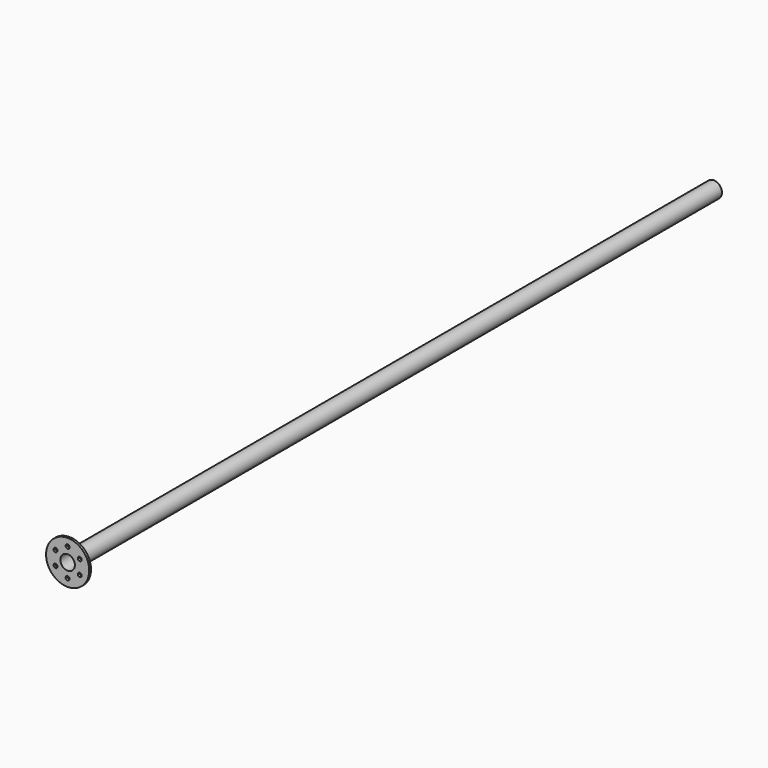
from build123d import *

# Parameters (mm, degrees)
F0_R            = 18.25
F0_R_2          = 16.25
F1_DEPTH        = 1800
F2_R            = 48.25
F2_R_2          = 18.25
F2_R_3          = 16.25
F3_DEPTH        = 5
F5_D            = 8.8
F5_COPIES_COUNT = 6


# Not quite as in the source:
# - a pattern or mirror of a feature is missing from the dataset's text; its kind, count and spacing are read off the source's solid


with BuildPart() as f1:
    # F0 (on Front) → F1 (new body)
    with BuildSketch(Plane.XZ):
        Circle(F0_R)
        Circle(F0_R_2, mode=Mode.SUBTRACT)
    extrude(amount=F1_DEPTH)

    # F2 (on face) → F3 (join)
    with BuildSketch(Plane.XZ.offset(1800)):
        Circle(F2_R)
        Circle(F2_R_2, mode=Mode.SUBTRACT)
        Circle(F2_R_2)
        Circle(F2_R_3, mode=Mode.SUBTRACT)
    extrude(amount=F3_DEPTH)

    # F5 (through all)
    with Locations(Plane.XZ.offset(1805)):
        with Locations((0, 31.25)):
            f5 = Hole(F5_D / 2)

    # F5_copies: F5 ×6 about axis
    f5_copies_axis = Axis((0, 0, 0), (0, 1, 0))
    for i in range(1, F5_COPIES_COUNT):
        add(f5.rotate(f5_copies_axis, i * 360 / F5_COPIES_COUNT), mode=Mode.SUBTRACT)


solid = f1.part
